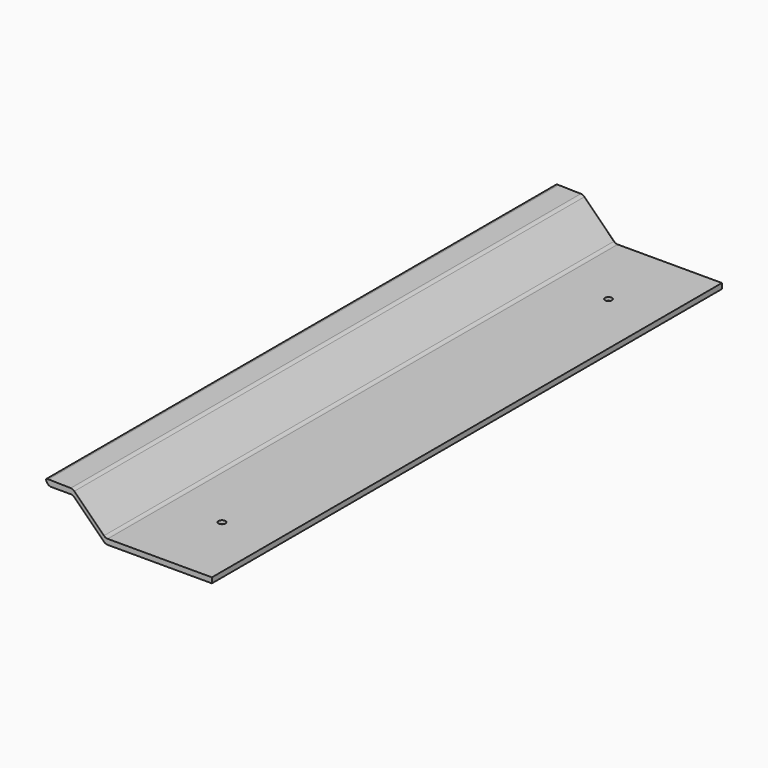
from build123d import *

# Parameters (mm, degrees)
F1_DEPTH       = 600
F2_R           = 5
F3_R           = 5
F4_T1_DEPTH    = 611.3695297687
F5_SIZE        = 1
F7_D           = 2.5
F7_CBORE_D     = 6.5
F7_CBORE_DEPTH = 3


# Not quite as in the source:
# - a fillet or chamfer that OpenCascade refuses, or shapes differently, is made with other operations: its cross-section is extruded or revolved along the edge and cut away or added


with BuildPart() as f1:
    # F0 (on Front) → F1 (new body)
    with BuildSketch(Plane.XZ):
        Polygon((-100, 12.6136353192), (0, 12.6136353192), (0, 17.5048394176), (0, 17.6136353192), (-100, 17.6136353192), (-125.63551, 43.2491453192), (-130.63551, 48.2491453192), (-155.818130374, 48.7903356552), (-155.818130374, 43.2491453192), (-130.63551, 43.2491453192), align=None)
    extrude(amount=F1_DEPTH)

    # F2
    f2_edges = [f1.edges().sort_by_distance(p)[0] for p in [
        (-130.63551, -300, 48.249145),
        (-100, -300, 17.613635),
    ]]
    fillet(f2_edges, radius=F2_R)

    # F3
    f3_edges = [f1.edges().sort_by_distance(p)[0] for p in [
        (-130.63551, -300, 43.249145),
        (-100, -300, 12.613635),
        (-155.81813, -300, 43.249145),
    ]]
    fillet(f3_edges, radius=F3_R)

    # F4: fillet of radius 5 on 1 edges, made by hand

    # F4_s2 → F4_t1 (cut)
    with BuildSketch(Plane.XZ.offset(-5.6847648844)):
        with BuildLine():
            ThreePointArc((-155.818130374, 48.2491453192), (-154.7104681905, 48.6293523426), (-153.5447493368, 48.7414792682))
            Line((-153.5447493368, 48.7414792682), (-155.818130374, 48.7903356552))
            Line((-155.818130374, 48.7903356552), (-155.818130374, 48.2491453192))
        make_face()
    extrude(amount=F4_T1_DEPTH, mode=Mode.SUBTRACT)

    # F5
    f5_edges = [f1.edges().sort_by_distance(p)[0] for p in [
        (-48.964466, 0, 17.613635),
        (-48.964466, 0, 12.613635),
        (-115.317755, 0, 27.93139),
        (-130.793161, 0, 42.868543),
        (-141.762354, 0, 43.249145),
        (-154.353664, 0, 44.713611),
        (-143.094103, 0, 48.516888),
        (-130.787949, 0, 47.892026),
        (-154.710468, 0, 48.629352),
        (-99.842349, 0, 12.994238),
        (-99.842349, 0, 17.994238),
        (-115.339908, 0, 32.953543),
        (0, 0, 15.113635),
    ]]
    chamfer(f5_edges, length=F5_SIZE)

    # F7 (through all)
    with Locations(Plane.XY.offset(17.6136353192)):
        with Locations((-48.9644660941, -73), (-48.9644660941, -527)):
            CounterBoreHole(F7_D / 2, F7_CBORE_D / 2, F7_CBORE_DEPTH)


solid = f1.part
